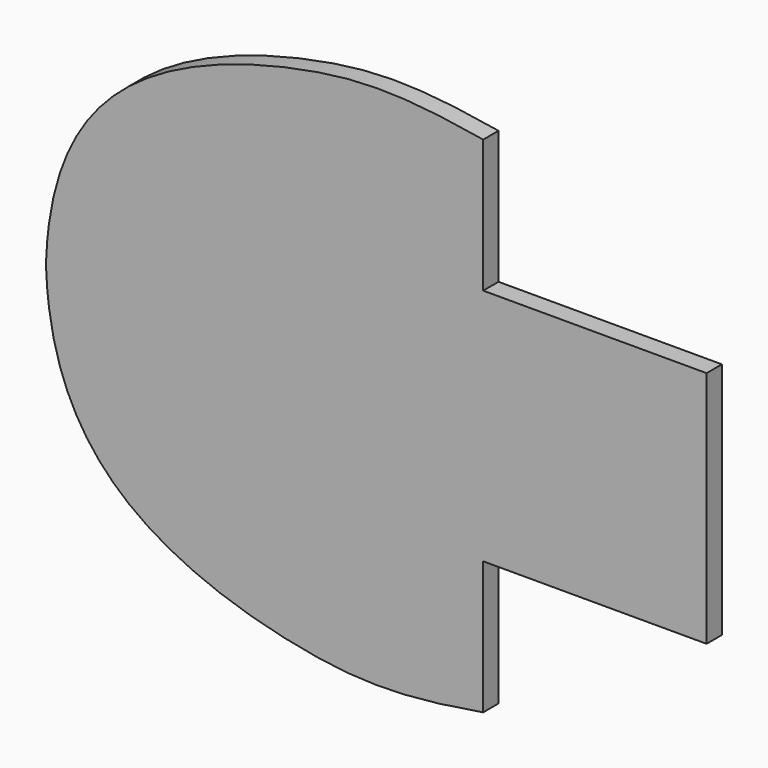
from build123d import *

# Parameters (mm, degrees)
F1_DEPTH    = 18
F2_T1_DEPTH = 18


# Not quite as in the source:
# - a fillet or chamfer that OpenCascade refuses, or shapes differently, is made with other operations: its cross-section is extruded or revolved along the edge and cut away or added


with BuildPart() as f1:
    # F0 (on Front) → F1 (new body)
    with BuildSketch(Plane.XZ):
        with BuildLine():
            Line((295, -217), (-326, -217))
            add(Edge.make_bspline(
                [(85, -454), (9.4357049053, -467.1385897042), (-72.818934134, -466.1104352643), (-260.3771381726, -409.0142413584), (-323.4175443649, -304.8886355162), (-326, -217)],
                knots=[0, 0, 0, 0, 0.3230188863, 0.6489287258, 1, 1, 1, 1], degree=3))
            Line((85, -454), (85, -329))
            Line((85, -329), (295, -329))
            Line((295, -329), (295, -217))
        make_face()
        with BuildLine():
            add(Edge.make_bspline(
                [(85, 20), (9.4357049053, 33.1385897042), (-72.818934134, 32.1104352643), (-260.3771381726, -24.9857586416), (-323.4175443649, -129.1113644838), (-326, -217)],
                knots=[0, 0, 0, 0, 0.3230188863, 0.6489287258, 1, 1, 1, 1], degree=3))
            Line((-326, -217), (295, -217))
            Line((295, -217), (295, -105))
            Line((295, -105), (85, -105))
            Line((85, -105), (85, 20))
        make_face()
    extrude(amount=F1_DEPTH)

    # F2: fillet of radius 100 on 1 edges, made by hand

    # F2_s2 → F2_t1 (cut)
    with BuildSketch(Plane.XZ):
        with BuildLine():
            ThreePointArc((-325.8594220148, -221.0337656795), (-325.9408114638, -217), (-325.8594220148, -212.9662343205))
            Line((-325.8594220148, -212.9662343205), (-327.8577942258, -212.8855590069))
            ThreePointArc((-327.8577942258, -212.8855590069), (-327.9340315871, -214.9132915531), (-327.999137182, -216.9412588095))
            Line((-327.999137182, -216.9412588095), (-327.999137182, -217.0587411905))
            ThreePointArc((-327.999137182, -217.0587411905), (-327.9340315871, -219.0867084469), (-327.8577942258, -221.1144409931))
            Line((-327.8577942258, -221.1144409931), (-325.8594220148, -221.0337656795))
        make_face()
    extrude(amount=F2_T1_DEPTH, mode=Mode.SUBTRACT)


solid = f1.part
